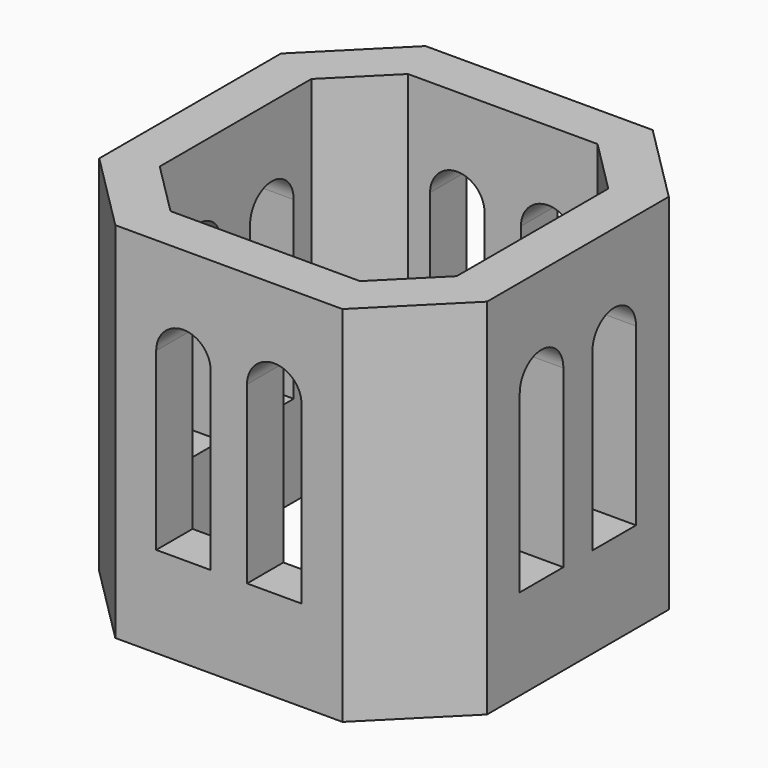
from build123d import *

# Parameters (mm, degrees)
F1_DEPTH = 4000
F3_W     = 600
F3_H     = 1250
F3_W_2   = 1250
F3_H_2   = 600
F4_DEPTH = 2230
F5_R     = 299.99999


# Not quite as in the source:
# - a fillet or chamfer is up to 0.001 mm smaller than in the source, because OpenCascade refuses the exact size


with BuildPart() as f1:
    # F0 (on Top) → F1 (new body)
    with BuildSketch(Plane.XY):
        Polygon((1250, 2133.8834764832), (-1250, 2133.8834764832), (-2133.8834764832, 1250), (-2133.8834764832, -1250), (-1250, -2133.8834764832), (1250, -2133.8834764832), (2133.8834764832, -1250), (2133.8834764832, 1250), align=None)
        Polygon((1633.8834764832, -1042.8932188135), (1042.8932188135, -1633.8834764832), (-1042.8932188135, -1633.8834764832), (-1633.8834764832, -1042.8932188135), (-1633.8834764832, 1042.8932188135), (-1042.8932188135, 1633.8834764832), (1042.8932188135, 1633.8834764832), (1633.8834764832, 1042.8932188135), align=None, mode=Mode.SUBTRACT)
    extrude(amount=F1_DEPTH)

    # F3 (on offset) → F4 (cut)
    with BuildSketch(Plane(origin=(0, 0, 1000), x_dir=(1, 0, 0), z_dir=(0, 0, -1))):
        with Locations((-500, -1875)):
            Rectangle(F3_W, F3_H)
        with Locations((500, -1875)):
            Rectangle(F3_W, F3_H)
        with Locations((-1875, 500)):
            Rectangle(F3_W_2, F3_H_2)
        with Locations((-1875, -500)):
            Rectangle(F3_W_2, F3_H_2)
        with Locations((500, 1875)):
            Rectangle(F3_W, F3_H)
        with Locations((-500, 1875)):
            Rectangle(F3_W, F3_H)
        with Locations((1875, -500)):
            Rectangle(F3_W_2, F3_H_2)
        with Locations((1875, 500)):
            Rectangle(F3_W_2, F3_H_2)
    extrude(amount=-F4_DEPTH, mode=Mode.SUBTRACT)

    # F5 (radius 300 in the source; OpenCascade refuses exactly that, so slightly less here)
    f5_edges = [f1.edges().sort_by_distance(p)[0] for p in [
        (-1883.883476, -800, 3230),
        (-1883.883476, -200, 3230),
        (-1883.883476, 800, 3230),
        (-1883.883476, 200, 3230),
        (-200, 1883.883476, 3230),
        (800, 1883.883476, 3230),
        (-800, 1883.883476, 3230),
        (200, 1883.883476, 3230),
        (1883.883476, 200, 3230),
        (1883.883476, -800, 3230),
        (1883.883476, 800, 3230),
        (1883.883476, -200, 3230),
        (200, -1883.883476, 3230),
        (-800, -1883.883476, 3230),
        (800, -1883.883476, 3230),
        (-200, -1883.883476, 3230),
    ]]
    fillet(f5_edges, radius=F5_R)


solid = f1.part
